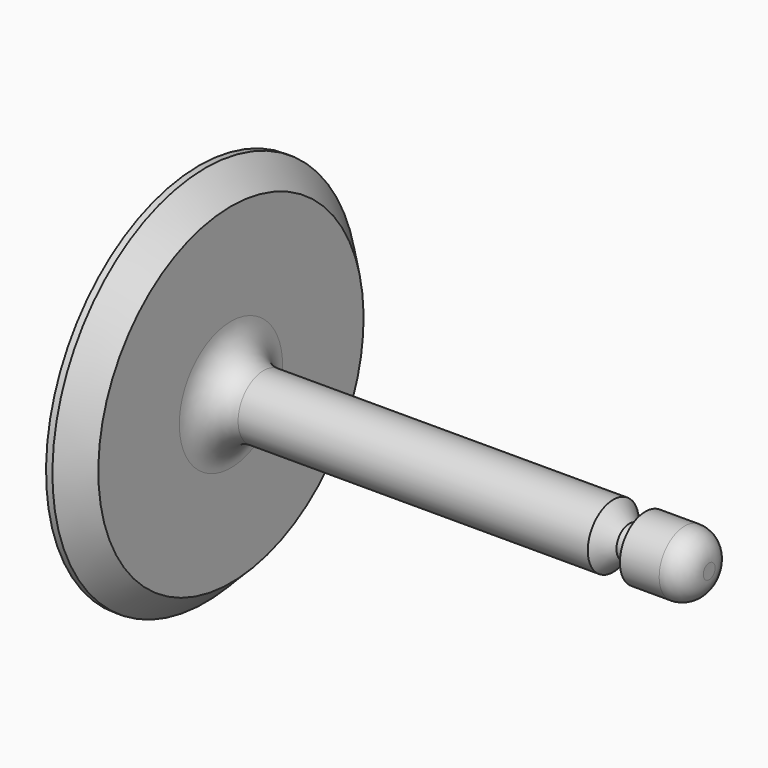
from build123d import *

# Parameters (mm, degrees)
F2_R        = 3.2512
F3_SIZE2    = 2.54
F3_SIZE     = 2.54
F4_S5_R     = 1.5875
F4_T6_DEPTH = 6
F5_R        = 2.4384


# Not quite as in the source:
# - a fillet or chamfer that OpenCascade refuses, or shapes differently, is made with other operations: its cross-section is extruded or revolved along the edge and cut away or added


with BuildPart() as f1:
    # F0 (on Front) → F1 (revolve)
    with BuildSketch(Plane.XZ):
        Polygon((-50.8, 0), (0, 0), (0, 3.175), (-6.35, 3.175), (-6.35, 1.5875), (-7.9502, 1.5875), (-7.9502, 3.175), (-47.625, 3.175), (-47.625, 19.05), (-50.8, 19.05), align=None)
    revolve(axis=Axis((-25.4, 0, 0), (1, 0, 0)))

    # F2
    f2_edges = [f1.edges().sort_by_distance(p)[0] for p in [
        (-47.625, 0, -3.175),
    ]]
    fillet(f2_edges, radius=F2_R)

    # F3
    f3_edges = [f1.edges().sort_by_distance(p)[0] for p in [
        (-47.625, 0, -6.4262),
        (-47.625, 0, -19.05),
    ]]
    chamfer(f3_edges, length=F3_SIZE, length2=F3_SIZE2)

    # F4: chamfer of 1.6002 on 1 edges, made by hand


with BuildPart() as f4_tool2:
    # F4_s3 → F4_t4 (revolve)
    with BuildSketch(Plane.XZ):
        Polygon((-9.5504, 3.175), (-7.9502, 1.5748), (-7.9502, 3.175), align=None)
    revolve(axis=Axis((-7.9502, 0, 0), (1, 0, 0)))

    # F4_s5 → F4_t6 (cut, symmetric)
    with BuildSketch(Plane.YZ.offset(-8.8)):
        Circle(F4_S5_R)
    extrude(amount=F4_T6_DEPTH, both=True, mode=Mode.SUBTRACT)


with BuildPart() as f1_1:
    add(f1.part)

    # F4_t1: cut F4_tool2
    add(f4_tool2.part, mode=Mode.SUBTRACT)

    # F5
    f5_edges = [f1_1.edges().sort_by_distance(p)[0] for p in [
        (0, 0, -3.175),
    ]]
    fillet(f5_edges, radius=F5_R)


solid = f1_1.part
